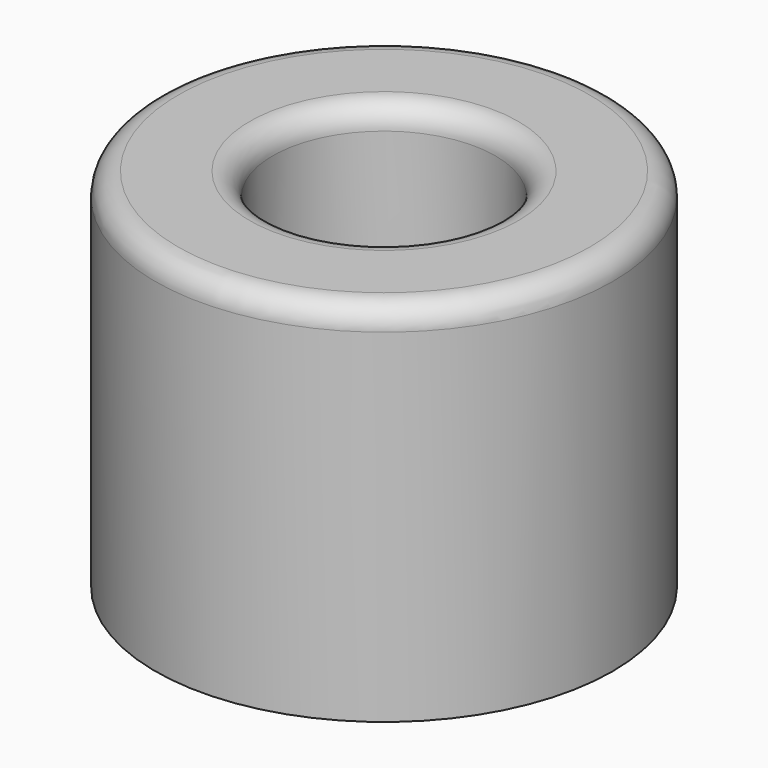
from build123d import *

# Parameters (mm, degrees)
F0_R           = 10
F1_DEPTH       = 16
F3_D           = 5.5
F3_CBORE_D     = 9.75
F3_CBORE_DEPTH = 5.5
F4_R           = 1


with BuildPart() as f1:
    # F0 (on Top) → F1 (new body)
    with BuildSketch(Plane.XY):
        Circle(F0_R)
    extrude(amount=F1_DEPTH)

    # F3 (through all)
    with Locations(Plane.XY.offset(16)):
        with Locations((0, 0)):
            CounterBoreHole(F3_D / 2, F3_CBORE_D / 2, F3_CBORE_DEPTH)

    # F4
    f4_edges = [f1.edges().sort_by_distance(p)[0] for p in [
        (-10, 0, 16),
        (-4.875, 0, 16),
    ]]
    fillet(f4_edges, radius=F4_R)


solid = f1.part
